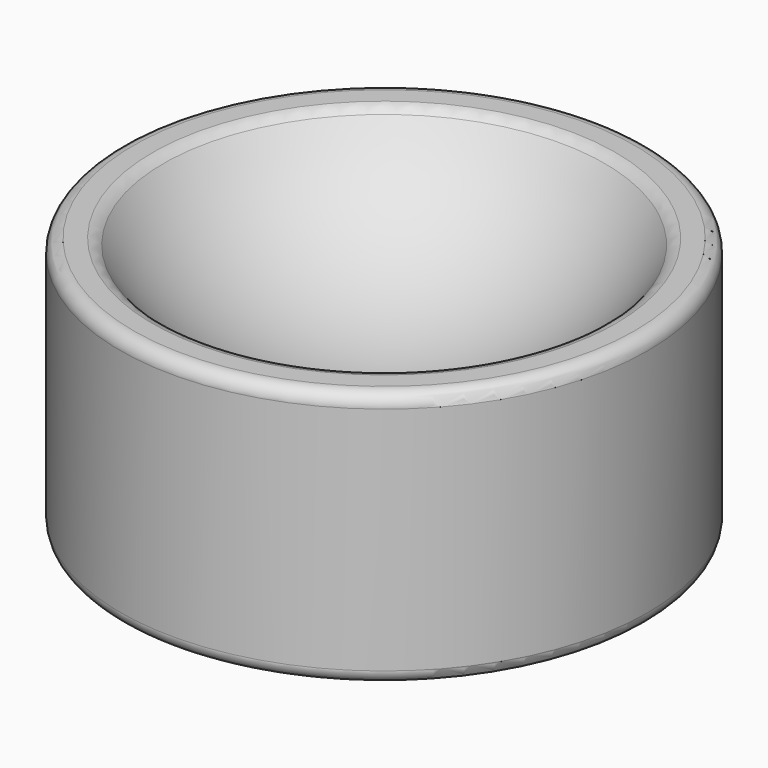
from build123d import *

# Parameters (mm, degrees)
F2_R     = 2.5
F3_DEPTH = 1
F4_R     = 2.5
F5_DEPTH = 4
F6_R     = 0.49999
F7_R     = 0.5


# Not quite as in the source:
# - a fillet or chamfer is up to 0.001 mm smaller than in the source, because OpenCascade refuses the exact size


with BuildPart() as f1:
    # F0 (on Front) → F1 (revolve)
    with BuildSketch(Plane.XZ):
        with BuildLine():
            ThreePointArc((8.5, -5.2678268764), (4.8642435813, -8.7372269275), (0, -10))
            Line((0, -10), (0, -15))
            Line((0, -15), (10, -15))
            Line((10, -15), (10, -5.2678268764))
            Line((10, -5.2678268764), (8.5, -5.2678268764))
        make_face()
    revolve(axis=Axis((0, 0, -12.5), (0, 0, 1)))

    # F2 (on face) → F3 (cut)
    with BuildSketch(Plane(origin=(0, 0, -15), x_dir=(1, 0, 0), z_dir=(0, 0, -1))):
        Circle(F2_R)
    extrude(amount=-F3_DEPTH, mode=Mode.SUBTRACT)

    # F4 (on face) → F5 (cut)
    with BuildSketch(Plane(origin=(0, 0, -15), x_dir=(1, 0, 0), z_dir=(0, 0, -1))):
        with Locations((-5.1961524227, 3)):
            Circle(F4_R)
        with Locations((0, 6)):
            Circle(F4_R)
        with Locations((5.1961524227, 3)):
            Circle(F4_R)
        with Locations((5.1961524227, -3)):
            Circle(F4_R)
        with Locations((0, -6)):
            Circle(F4_R)
        with Locations((-5.1961524227, -3)):
            Circle(F4_R)
    extrude(amount=-F5_DEPTH, mode=Mode.SUBTRACT)

    # F6 (radius 0.5 in the source; OpenCascade refuses exactly that, so slightly less here)
    f6_edges = [f1.edges().sort_by_distance(p)[0] for p in [
        (2.696152, 3, -15),
        (-2.5, 6, -15),
        (-7.696152, 3, -15),
        (-7.696152, -3, -15),
        (-2.5, -6, -15),
        (2.696152, -3, -15),
        (2.696152, 3, -11),
        (-2.5, 6, -11),
        (-7.696152, 3, -11),
        (-7.696152, -3, -11),
        (-2.5, -6, -11),
        (2.696152, -3, -11),
    ]]
    fillet(f6_edges, radius=F6_R)

    # F7
    f7_edges = [f1.edges().sort_by_distance(p)[0] for p in [
        (-10, 0, -15),
        (-10, 0, -5.267827),
        (-8.5, 0, -5.267827),
    ]]
    fillet(f7_edges, radius=F7_R)


solid = f1.part
